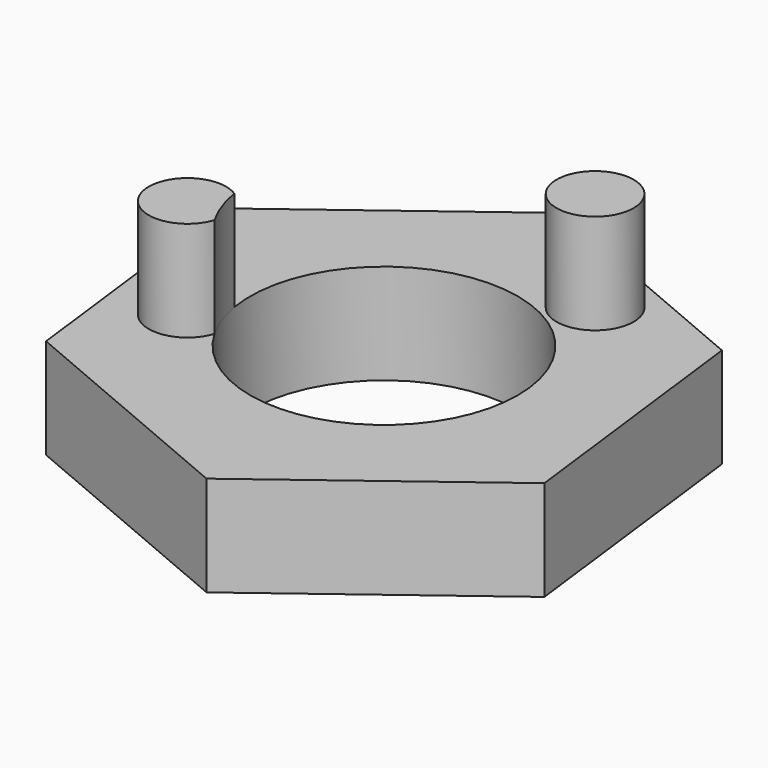
from build123d import *

# Parameters (mm, degrees)
F0_R     = 33.4292406747
F1_DEPTH = 25
F2_R     = 9.6236756303
F3_DEPTH = 25


# Not quite as in the source:
# - after a boolean that leaves OpenCascade's solid faulty, fix() repairs it


with BuildPart() as f1:
    # F0 (on Top) → F1 (new body)
    with BuildSketch(Plane.XY):
        Polygon((-8.0187594833, 61.3087737227), (-60.6567287502, 21.6589621043), (-52.6379692669, -43.7517622936), (8.0187594833, -69.5126750732), (60.6567287502, -29.8628634548), (52.6379692669, 35.5478609431), align=None)
        with Locations((0, -4.1019506752)):
            Circle(F0_R, mode=Mode.SUBTRACT)
    extrude(amount=F1_DEPTH)

    # F2 (on face) → F3 (join)
    with BuildSketch(Plane.XY.offset(25)):
        with BuildLine():
            ThreePointArc((-28.942967923, -20.8297341476), (-31.4616986723, -15.4013156461), (-32.9722113693, -9.6107989674))
            ThreePointArc((-32.9722113693, -9.6107989674), (-47.2113068424, -21.0577353047), (-28.942967923, -20.8297341476))
        make_face()
        with Locations((22.0662225038, 34.1823846102)):
            Circle(F2_R)
    extrude(amount=F3_DEPTH)

    add(f1.part.fix(), mode=Mode.REPLACE)


solid = f1.part
